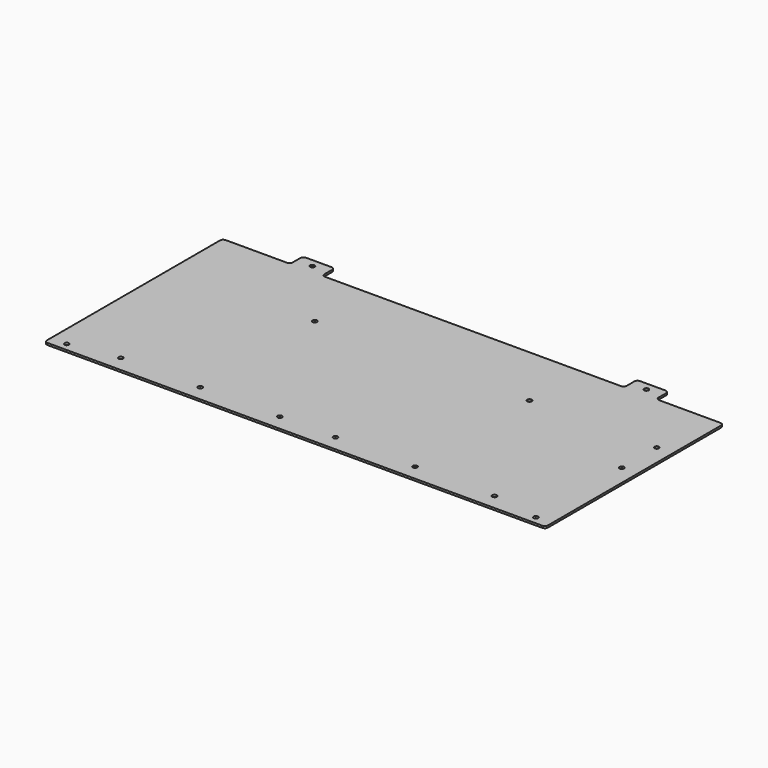
from build123d import *

# Parameters (mm, degrees)
F0_W     = 107.95
F0_H     = 355.6
F0_W_2   = 50.8
F0_H_2   = 25.4
F1_DEPTH = 3.175
F2_D     = 7.1374
F3_R     = 5.08
F5_D     = 7.1374


# Not quite as in the source:
# - a feature names something its author has since deleted; it is built from what else it names


with BuildPart() as f1:
    # F0 (on Top) → F1 (new body)
    with BuildSketch(Plane.XY):
        with Locations((53.975, 177.8)):
            Rectangle(F0_W, F0_H)
        Polygon((107.95, 355.6), (107.95, 0), (400.05, 0), (400.05, 355.6), (158.75, 355.6), align=None)
        with Locations((133.35, 368.3)):
            Rectangle(F0_W_2, F0_H_2)
        Polygon((400.05, 355.6), (400.05, 0), (692.15, 0), (692.15, 355.6), (641.35, 355.6), align=None)
        with Locations((746.125, 177.8)):
            Rectangle(F0_W, F0_H)
        with Locations((666.75, 368.3)):
            Rectangle(F0_W_2, F0_H_2)
    extrude(amount=F1_DEPTH)

    # F2 (through all)
    with Locations(Plane(origin=(0, 0, 0), x_dir=(1, 0, 0), z_dir=(0, 0, -1))):
        with Locations((133.35, -368.3), (666.75, -368.3), (25.4, -12.7), (774.7, -12.7)):
            Hole(F2_D / 2)

    # F3
    f3_edges = [f1.edges().sort_by_distance(p)[0] for p in [
        (0, 355.6, 1.5875),
        (107.95, 355.6, 1.5875),
        (107.95, 381, 1.5875),
        (158.75, 381, 1.5875),
        (158.75, 355.6, 1.5875),
        (692.15, 355.6, 1.5875),
        (692.15, 381, 1.5875),
        (641.35, 381, 1.5875),
        (641.35, 355.6, 1.5875),
        (800.1, 355.6, 1.5875),
        (800.1, 0, 1.5875),
        (0, 0, 1.5875),
    ]]
    fillet(f3_edges, radius=F3_R)

    # F5 (through all)
    with Locations(Plane.XY.offset(3.175)):
        with Locations((571.5, 254), (774.7, 254), (444.5, 25.4), (571.5, 25.4), (698.5, 25.4), (774.7, 184.15), (101.6, 25.4), (228.6, 25.4), (355.6, 25.4), (228.6, 254)):
            Hole(F5_D / 2)


solid = f1.part
